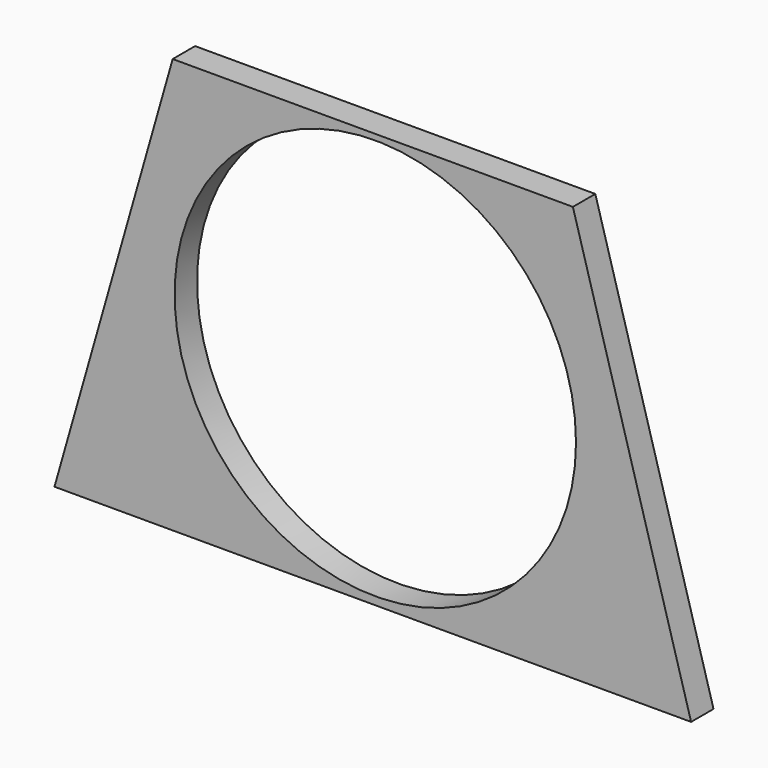
from build123d import *

# Parameters (mm, degrees)
F0_R     = 22.733
F1_DEPTH = 1.5875


# Not quite as in the source:
# - a feature names something its author has since deleted; it is built from what else it names


with BuildPart() as f1:
    # F0 (on Front) → F1 (new body, symmetric)
    with BuildSketch(Plane.XZ):
        Polygon((22.3805892097, 23.3813975786), (-22.9507907903, 23.3813975786), (-36.3404007903, -23.6231935325), (35.7701992097, -23.6231935325), align=None)
        Circle(F0_R, mode=Mode.SUBTRACT)
    extrude(amount=F1_DEPTH, both=True)


solid = f1.part
